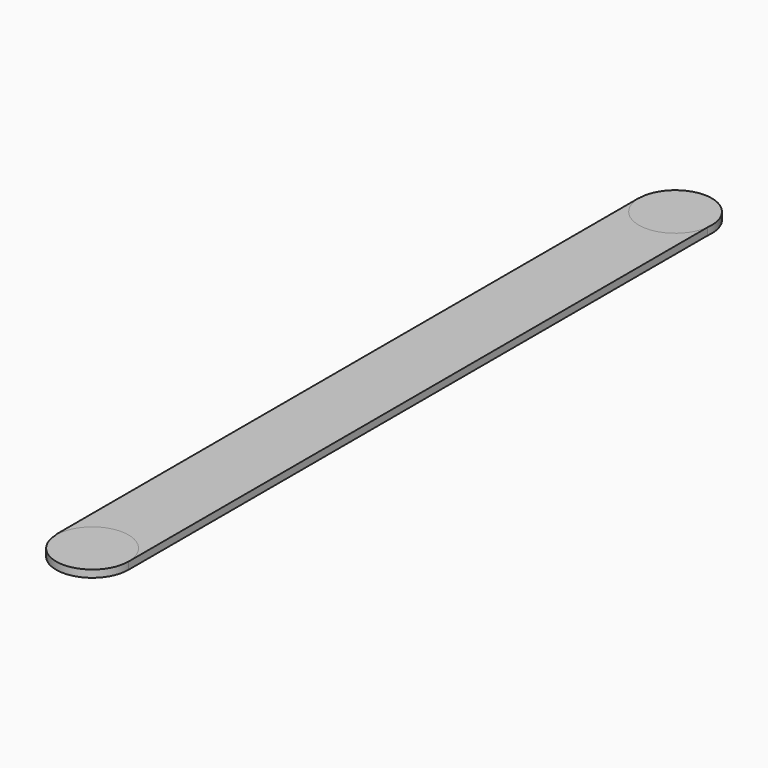
from build123d import *

# Parameters (mm, degrees)
F0_W     = 5.08
F0_H     = 50.8
F3_DEPTH = 0.508
F1_R     = 2.5422270568
F1_R_2   = 2.5183658608


with BuildPart() as f3:
    # F0 (on Top) → F3 (new body)
    with BuildSketch(Plane.XY):
        with Locations((-54.4140953571, 39.7249583329)):
            Rectangle(F0_W, F0_H)
    extrude(amount=F3_DEPTH)


with BuildPart() as f3b:
    # F1 (on Top) → F3, piece 2 (new body)
    with BuildSketch(Plane.XY):
        with Locations((-54.3948672712, 65.1251375675)):
            Circle(F1_R)
    extrude(amount=F3_DEPTH)


with BuildPart() as f3c:
    # F1 (on Top) → F3, piece 3 (new body)
    with BuildSketch(Plane.XY):
        with Locations((-54.3948672712, 14.3131716177)):
            Circle(F1_R_2)
    extrude(amount=F3_DEPTH)


solid = Compound([f3.part, f3b.part, f3c.part])
